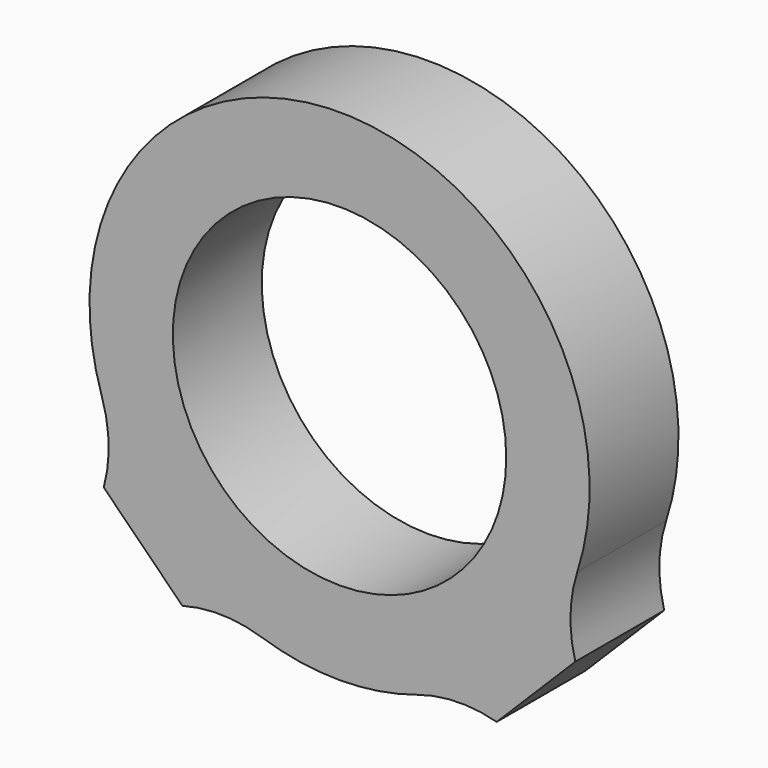
from build123d import *

# Parameters (mm, degrees)
F1_DEPTH    = 2
F2_T1_DEPTH = 4


# Not quite as in the source:
# - a fillet or chamfer that OpenCascade refuses, or shapes differently, is made with other operations: its cross-section is extruded or revolved along the edge and cut away or added


with BuildPart() as f1:
    # F0 (on Front) → F1 (new body, symmetric)
    with BuildSketch(Plane.XZ):
        with BuildLine():
            ThreePointArc((-4.7906232606, -7.6190503854), (-2.4928444127, -8.6478741165), (0, -9))
            ThreePointArc((0, -9), (2.4928444127, -8.6478741165), (4.7906232606, -7.6190503854))
            Line((4.7906232606, -7.6190503854), (5.6568542495, -8.4852813742))
            Line((5.6568542495, -8.4852813742), (8.4852813742, -5.6568542495))
            Line((8.4852813742, -5.6568542495), (7.6190503854, -4.7906232606))
            ThreePointArc((7.6190503854, -4.7906232606), (0, 9), (-7.6190503854, -4.7906232606))
            Line((-7.6190503854, -4.7906232606), (-8.4852813742, -5.6568542495))
            Line((-8.4852813742, -5.6568542495), (-5.6568542495, -8.4852813742))
            Line((-5.6568542495, -8.4852813742), (-4.7906232606, -7.6190503854))
        make_face()
        with BuildLine():
            ThreePointArc((0, -6), (-4.2426406871, 4.2426406871), (6, 0))
            ThreePointArc((6, 0), (4.2426406871, -4.2426406871), (0, -6))
        make_face(mode=Mode.SUBTRACT)
    extrude(amount=F1_DEPTH, both=True)

    # F2: fillet of radius 5 on 4 edges, made by hand

    # F2_s2 → F2_t1 (join)
    with BuildSketch(Plane.XZ.offset(-2)):
        with BuildLine():
            ThreePointArc((8.5560838448, -2.7916714064), (8.3109896839, -4.2190810375), (8.4852813742, -5.6568542495))
            Line((8.4852813742, -5.6568542495), (7.6190503854, -4.7906232606))
            ThreePointArc((7.6190503854, -4.7906232606), (8.149091604, -3.8199877003), (8.5560838448, -2.7916714064))
        make_face()
        with BuildLine():
            ThreePointArc((5.6568542495, -8.4852813742), (4.2190810375, -8.3109896839), (2.7916714064, -8.5560838448))
            ThreePointArc((2.7916714064, -8.5560838448), (3.8199877003, -8.149091604), (4.7906232606, -7.6190503854))
            Line((4.7906232606, -7.6190503854), (5.6568542495, -8.4852813742))
        make_face()
        with BuildLine():
            ThreePointArc((-2.7916714064, -8.5560838448), (-4.2190810375, -8.3109896839), (-5.6568542495, -8.4852813742))
            Line((-5.6568542495, -8.4852813742), (-4.7906232606, -7.6190503854))
            ThreePointArc((-4.7906232606, -7.6190503854), (-3.8199877003, -8.149091604), (-2.7916714064, -8.5560838448))
        make_face()
        with BuildLine():
            ThreePointArc((-8.4852813742, -5.6568542495), (-8.3109896839, -4.2190810375), (-8.5560838448, -2.7916714064))
            ThreePointArc((-8.5560838448, -2.7916714064), (-8.149091604, -3.8199877003), (-7.6190503854, -4.7906232606))
            Line((-7.6190503854, -4.7906232606), (-8.4852813742, -5.6568542495))
        make_face()
    extrude(amount=F2_T1_DEPTH)


solid = f1.part
